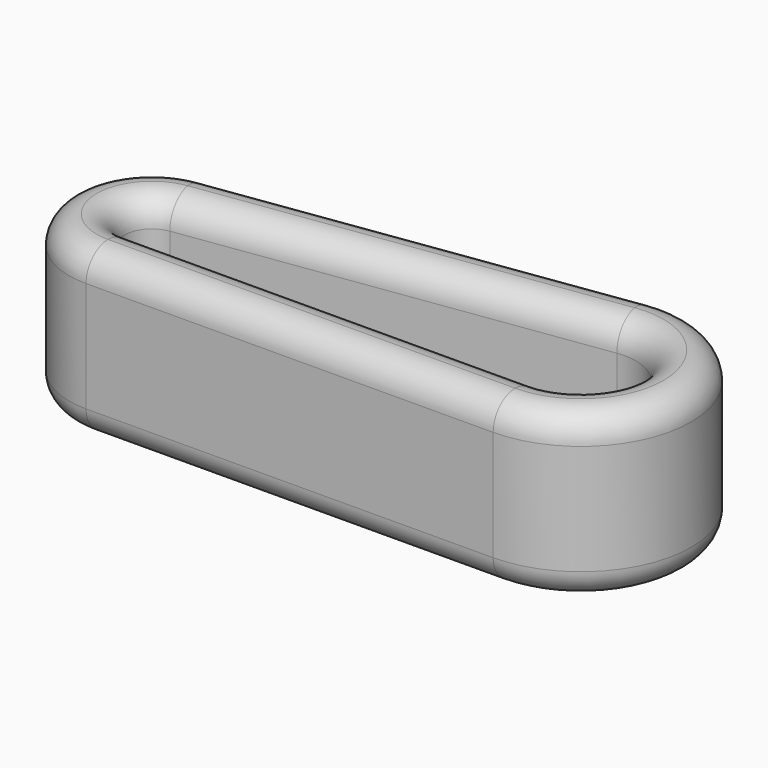
from build123d import *

# Parameters (mm, degrees)
F1_DEPTH = 30
F2_DEPTH = 25.4
F3_R     = 4.99999


# Not quite as in the source:
# - a fillet or chamfer is up to 0.001 mm smaller than in the source, because OpenCascade refuses the exact size


with BuildPart() as f1:
    # F0 (on Top) → F1 (new body)
    with BuildSketch(Plane.XY):
        with BuildLine():
            Line((34.7105600204, 69.6575524111), (-38.0615795526, 59.3297830847))
            ThreePointArc((-38.0615795526, 59.3297830847), (-50.9138983938, 43.3837240922), (-35.8768828371, 29.4787947456))
            Line((-35.8768828371, 29.4787947456), (37.6234889744, 29.8562346256))
            ThreePointArc((37.6234889744, 29.8562346256), (57.4674373389, 51.3158014327), (34.7105600204, 69.6575524111))
        make_face()
        with BuildLine():
            ThreePointArc((36.1156730696, 59.756761669), (47.4941117288, 50.5858861798), (37.5721375466, 39.8561027762))
            Line((37.5721375466, 39.8561027762), (-35.9282342649, 39.4786628962))
            ThreePointArc((-35.9282342649, 39.4786628962), (-40.9405727838, 44.1136393451), (-36.6564665034, 49.4289923426))
            Line((-36.6564665034, 49.4289923426), (36.1156730696, 59.756761669))
        make_face(mode=Mode.SUBTRACT)
    extrude(amount=F1_DEPTH)

    # F0 (on Top) → F2 (join)
    with BuildSketch(Plane.XY):
        with BuildLine():
            Line((34.7105600204, 69.6575524111), (-38.0615795526, 59.3297830847))
            ThreePointArc((-38.0615795526, 59.3297830847), (-50.9138983938, 43.3837240922), (-35.8768828371, 29.4787947456))
            Line((-35.8768828371, 29.4787947456), (37.6234889744, 29.8562346256))
            ThreePointArc((37.6234889744, 29.8562346256), (57.4674373389, 51.3158014327), (34.7105600204, 69.6575524111))
        make_face()
        with BuildLine():
            ThreePointArc((36.1156730696, 59.756761669), (47.4941117288, 50.5858861798), (37.5721375466, 39.8561027762))
            Line((37.5721375466, 39.8561027762), (-35.9282342649, 39.4786628962))
            ThreePointArc((-35.9282342649, 39.4786628962), (-40.9405727838, 44.1136393451), (-36.6564665034, 49.4289923426))
            Line((-36.6564665034, 49.4289923426), (36.1156730696, 59.756761669))
        make_face(mode=Mode.SUBTRACT)
    extrude(amount=F2_DEPTH)

    # F3 (radius 5 in the source; OpenCascade refuses exactly that, so slightly less here)
    f3_edges = [f1.edges().sort_by_distance(p)[0] for p in [
        (57.467437, 51.315801, 30),
        (-1.67551, 64.493668, 30),
        (-50.913898, 43.383724, 30),
        (0.873303, 29.667515, 30),
        (-40.940573, 44.113639, 30),
        (-0.270397, 54.592877, 30),
        (47.494112, 50.585886, 30),
        (0.821952, 39.667383, 30),
        (57.467437, 51.315801, 0),
        (-1.67551, 64.493668, 0),
        (-50.913898, 43.383724, 0),
        (0.873303, 29.667515, 0),
        (-40.940573, 44.113639, 0),
        (-0.270397, 54.592877, 0),
        (47.494112, 50.585886, 0),
        (0.821952, 39.667383, 0),
    ]]
    fillet(f3_edges, radius=F3_R)


solid = f1.part
